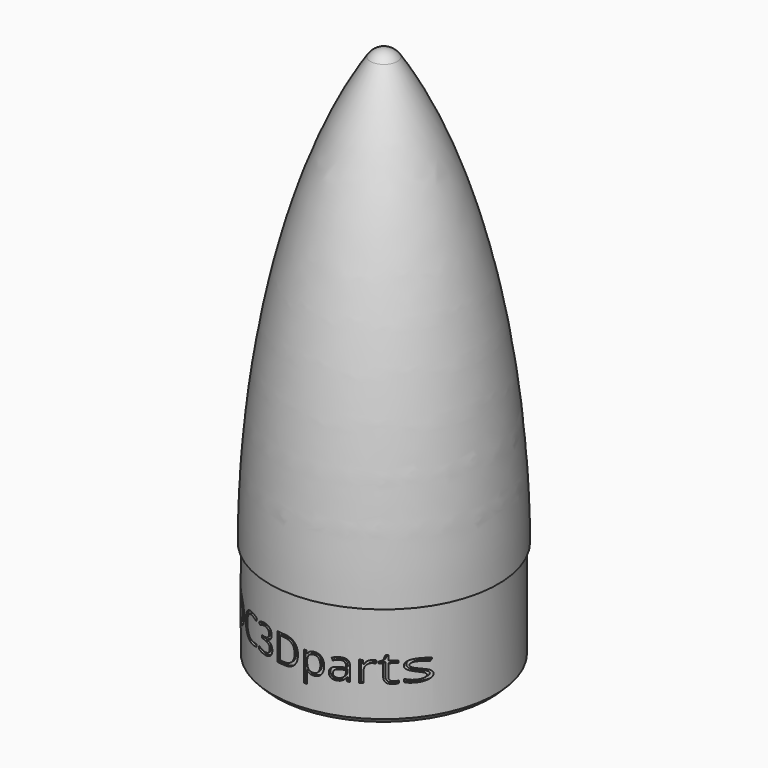
from build123d import *

# Parameters (mm, degrees)
F2_SIZE      = 1.5
F4_TEXT_SIZE = 11.1111111111
F5_DEPTH     = 40
F6_W         = 32
F6_H         = 32.6195528252


# Not quite as in the source:
# - Text() gives the source's letters only with a copy of the font that has no kerning and outlines rounded to 1/6400 em; it was checked with that copy


with BuildPart() as f1:
    # F0 (on Front) → F1 (revolve)
    with BuildSketch(Plane.XZ):
        with BuildLine():
            ThreePointArc((0, 57.9262248208), (-2.2146009548, 57.3697439286), (-3.903094682, 55.8325005173))
            add(Edge.make_bspline(
                [(-3.903094682, 55.8325005173), (-32.7962725337, 12.3108385484), (-33.3, -68.7499268014)],
                knots=[0.5734099772, 0.5734099772, 0.5734099772, 1.5951998253, 1.5951998253, 1.5951998253], degree=2, weights=[1, 0.8723072767, 1]))
            Line((-33.3, -68.7499268014), (-32.6, -68.7499268014))
            Line((-32.6, -68.7499268014), (-32.6, -98.7499268014))
            Line((-32.6, -98.7499268014), (0, -98.7499268014))
            Line((0, -98.7499268014), (0, -68.7499268014))
            Line((0, -68.7499268014), (0, 57.9262248208))
        make_face()
    revolve(axis=Axis((0, 0, 9.1068005099), (0, 0, 1)))

    # F2
    f2_edges = [f1.edges().sort_by_distance(p)[0] for p in [
        (32.6, 0, -98.749927),
    ]]
    chamfer(f2_edges, length=F2_SIZE)


with BuildPart() as f5:
    # F4 (on offset) → F5 (new body, through all)
    with BuildSketch(Plane.XZ.offset(40)):
        with Locations((-27.8669164908, -88.1734709394)):
            Text('DC3Dparts', F4_TEXT_SIZE, font='Open Sans', text_align=(TextAlign.LEFT, TextAlign.BOTTOM))
    extrude(amount=-F5_DEPTH)


with BuildPart() as f7:
    # F6 (on Front) → F7 (revolve)
    with BuildSketch(Plane.XZ):
        with Locations((-16, -87.7568681528)):
            Rectangle(F6_W, F6_H)
    revolve(axis=Axis((0, 0, -87.7568681528), (0, 0, -1)))


with BuildPart() as f5_1:
    add(f5.part)

    # F8: cut F7
    add(f7.part, mode=Mode.SUBTRACT)


with BuildPart() as f1_1:
    add(f1.part)

    # F9: cut F5
    add(f5_1.part, mode=Mode.SUBTRACT)


solid = f1_1.part
